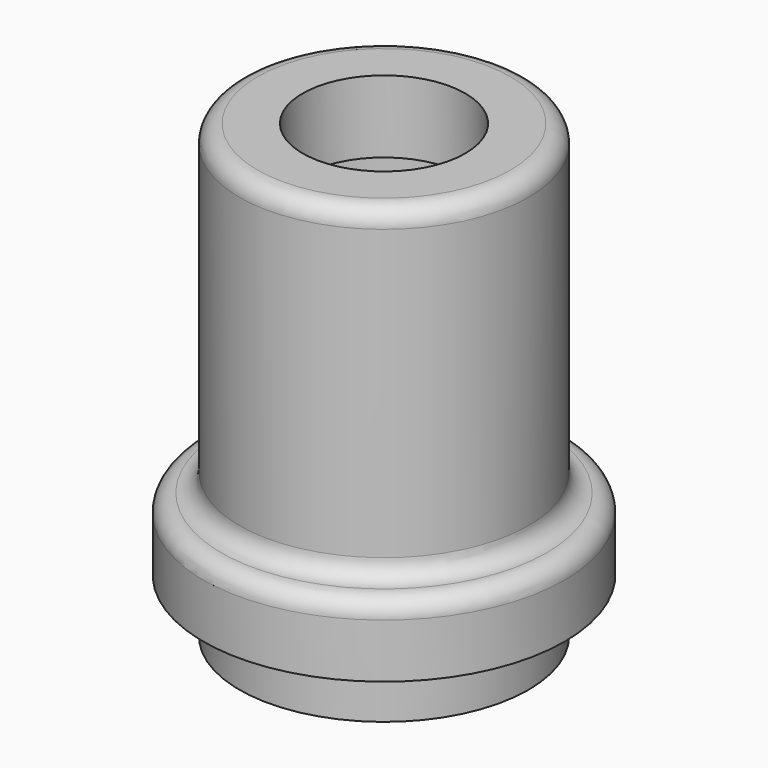
from build123d import *

# Parameters (mm, degrees)
F0_R          = 8
F0_R_2        = 6
F1_DEPTH      = 3
F0_R_3        = 10
F2_DEPTH      = 4
F3_DEPTH      = 25
F4_START      = 18
F4_DEPTH      = 4
F5_R          = 0.99999
F6_R          = 4.5
F7_DEPTH      = 25
F7_DEPTH_BACK = 25


# Not quite as in the source:
# - a fillet or chamfer is up to 0.001 mm smaller than in the source, because OpenCascade refuses the exact size


with BuildPart() as f1:
    # F0 (on Top) → F1 (new body)
    with BuildSketch(Plane.XY):
        Circle(F0_R)
        Circle(F0_R_2, mode=Mode.SUBTRACT)
    extrude(amount=-F1_DEPTH)

    # F0 (on Top) → F2 (join)
    with BuildSketch(Plane.XY):
        Circle(F0_R_3)
        Circle(F0_R, mode=Mode.SUBTRACT)
        Circle(F0_R)
        Circle(F0_R_2, mode=Mode.SUBTRACT)
    extrude(amount=F2_DEPTH)

    # F3 (add): a face of the model
    f3_faces = [f1.faces().sort_by_distance(p)[0] for p in [
        (-7.77372583, 0, -3),
    ]]
    extrude(f3_faces, amount=-F3_DEPTH)

    # F0 (on Top) → F4 (join)
    with BuildSketch(Plane.XY.offset(F4_START)):
        Circle(F0_R_2)
    extrude(amount=F4_DEPTH)

    # F5 (radius 1 in the source; OpenCascade refuses exactly that, so slightly less here)
    f5_edges = [f1.edges().sort_by_distance(p)[0] for p in [
        (-8, 0, 4),
        (-10, 0, 4),
        (-8, 0, 22),
    ]]
    fillet(f5_edges, radius=F5_R)

    # F6 (on face) → F7 (cut, two sides)
    with BuildSketch(Plane.XY.offset(22)) as f7_sk:
        Circle(F6_R)
    extrude(amount=-F7_DEPTH, mode=Mode.SUBTRACT)
    extrude(f7_sk.sketch, amount=F7_DEPTH_BACK, mode=Mode.SUBTRACT)


solid = f1.part
